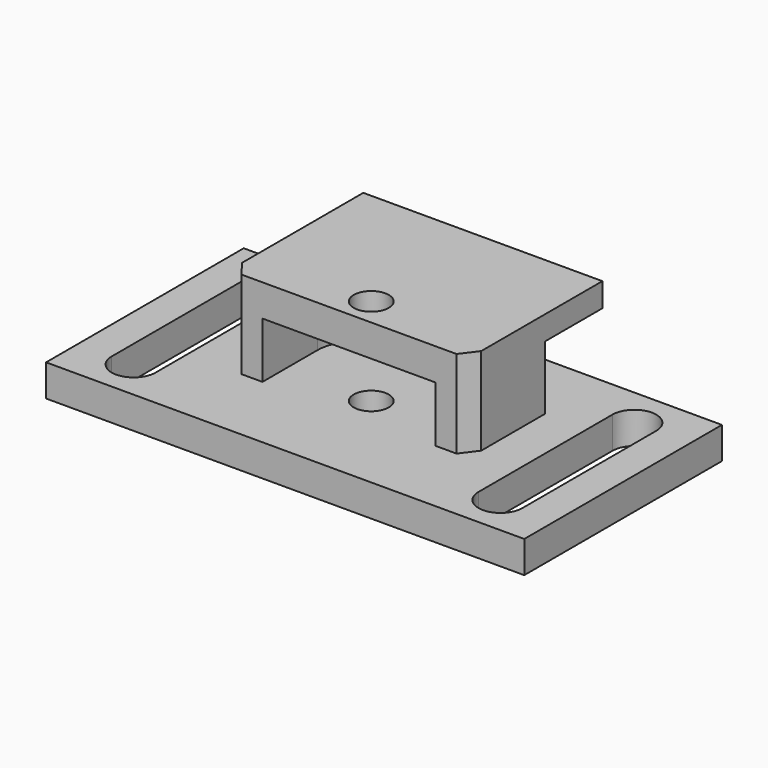
from build123d import *

# Parameters (mm, degrees)
F0_W         = 30
F0_H         = 26
F1_DEPTH     = 15
F3_SIZE2     = 2
F3_SIZE      = 1.5
F5_DEPTH     = 30.001
F6_SIZE      = 4
F2_W         = 21.7
F2_H         = 7
F7_DEPTH     = 12.5
F8_W         = 11
F8_H         = 7
F9_DEPTH     = 4
F10_W        = 30
F10_H        = 5
F11_DEPTH    = 15.001
F13_D        = 4.4
F15_DEPTH    = 4
F16_SIZE     = 3.49999
F17_T4_DEPTH = 26.4149188769
F18_SIZE     = 3.49999
F19_T4_DEPTH = 26.4149188769


# Not quite as in the source:
# - a fillet or chamfer that OpenCascade refuses, or shapes differently, is made with other operations: its cross-section is extruded or revolved along the edge and cut away or added
# - a fillet or chamfer is up to 0.001 mm smaller than in the source, because OpenCascade refuses the exact size


with BuildPart() as f1:
    # F0 (on Top) → F1 (new body)
    with BuildSketch(Plane.XY):
        Rectangle(F0_W, F0_H)
    extrude(amount=F1_DEPTH)

    # F3
    f3_edges = [f1.edges().sort_by_distance(p)[0] for p in [
        (-15, -13, 7.5),
        (15, -13, 7.5),
    ]]
    f3_side = f1.faces().sort_by_distance((0, -13, 7.5))[0]
    chamfer(f3_edges, length=F3_SIZE, length2=F3_SIZE2, reference=f3_side)

    # F4 (on face) → F5 (cut, through all)
    with BuildSketch(Plane(origin=(-15, 0, 0), x_dir=(0, -1, 0), z_dir=(-1, 0, 0))):
        Polygon((-13, 12), (-13, 0), (-8, 0), (-8, 4), (-3, 4), (-3, 12), align=None)
    extrude(amount=-F5_DEPTH, mode=Mode.SUBTRACT)

    # F6
    f6_edges = [f1.edges().sort_by_distance(p)[0] for p in [
        (-15, 3, 8),
        (15, 3, 8),
    ]]
    chamfer(f6_edges, length=F6_SIZE)

    # F2 (on face) → F7 (cut)
    with BuildSketch(Plane.XZ.offset(13)):
        with Locations((0, 7.5)):
            Rectangle(F2_W, F2_H)
    extrude(amount=-F7_DEPTH, mode=Mode.SUBTRACT)

    # F8 (on face) → F9 (cut)
    with BuildSketch(Plane(origin=(0, 3, 0), x_dir=(-1, 0, 0), z_dir=(0, 1, 0))):
        with Locations((0, 7.5)):
            Rectangle(F8_W, F8_H)
    extrude(amount=-F9_DEPTH, mode=Mode.SUBTRACT)

    # F10 (on face) → F11 (cut, through all)
    with BuildSketch(Plane.XY.offset(15)):
        with Locations((0, 10.5)):
            Rectangle(F10_W, F10_H)
    extrude(amount=-F11_DEPTH, mode=Mode.SUBTRACT)

    # F13 (through all)
    with Locations(Plane.XY.offset(15)):
        with Locations((0, -9.5)):
            Hole(F13_D / 2)

    # F14 (on face) → F15 (join)
    with BuildSketch(Plane(origin=(0, 0, 0), x_dir=(1, 0, 0), z_dir=(0, 0, -1))):
        with BuildLine():
            Line((30, 23), (-30, 23))
            Line((-30, 23), (-30, 11))
            Line((-30, 11), (-25.7624481171, 11))
            Line((-25.7624481171, 11), (-25.7624481171, 18))
            ThreePointArc((-25.7624481171, 18), (-23.0124481171, 20.75), (-20.2624481171, 18))
            Line((-20.2624481171, 18), (-20.2624481171, 11))
            Line((-20.2624481171, 11), (-15, 11))
            Line((-15, 11), (-13.5, 13))
            Line((-13.5, 13), (13.5, 13))
            Line((13.5, 13), (15, 11))
            Line((15, 11), (20.2624481171, 11))
            Line((20.2624481171, 11), (20.2624481171, 18))
            ThreePointArc((20.2624481171, 18), (23.0124481171, 20.75), (25.7624481171, 18))
            Line((25.7624481171, 18), (25.7624481171, 11))
            Line((25.7624481171, 11), (30, 11))
            Line((30, 11), (30, 23))
        make_face()
        with BuildLine():
            Line((-25.7624481171, 11), (-30, 11))
            Line((-30, 11), (-30, -8))
            Line((-30, -8), (-15, -8))
            Line((-15, -8), (-15, 11))
            Line((-15, 11), (-20.2624481171, 11))
            Line((-20.2624481171, 11), (-20.2624481171, -3))
            ThreePointArc((-20.2624481171, -3), (-23.0124481171, -5.75), (-25.7624481171, -3))
            Line((-25.7624481171, -3), (-25.7624481171, 11))
        make_face()
        with BuildLine():
            Line((30, -8), (30, 11))
            Line((30, 11), (25.7624481171, 11))
            Line((25.7624481171, 11), (25.7624481171, -3))
            ThreePointArc((25.7624481171, -3), (23.0124481171, -5.75), (20.2624481171, -3))
            Line((20.2624481171, -3), (20.2624481171, 11))
            Line((20.2624481171, 11), (15, 11))
            Line((15, 11), (15, -8))
            Line((15, -8), (30, -8))
        make_face()
    extrude(amount=-F15_DEPTH)

    # F16 (size 3.5 in the source; OpenCascade refuses exactly that, so slightly less here)
    f16_edges = [f1.edges().sort_by_distance(p)[0] for p in [
        (-5.5, -0.5, 7.5),
    ]]
    chamfer(f16_edges, length=F16_SIZE)

    # F17: fillet of radius 5 on 1 edges, made by hand


with BuildPart() as f17_tool2:
    # F17_s3 → F17_t4 (new body)
    with BuildSketch(Plane.XY.offset(20.7074594385)):
        with BuildLine():
            ThreePointArc((-8.99999, -0.5), (-10.3638647521, -2.2323966462), (-10.85, -4.3829837754))
            Line((-10.85, -4.3829837754), (-10.85, -0.5))
            Line((-10.85, -0.5), (-8.99999, -0.5))
        make_face()
    extrude(amount=-F17_T4_DEPTH)

    split(bisect_by=Plane.XY.offset(15), keep=Keep.BOTTOM)

    split(bisect_by=Plane.XY, keep=Keep.TOP)


with BuildPart() as f1_1:
    add(f1.part)

    # F17_t1: union F17_tool2
    add(f17_tool2.part)

    # F18 (size 3.5 in the source; OpenCascade refuses exactly that, so slightly less here)
    f18_edges = [f1_1.edges().sort_by_distance(p)[0] for p in [
        (5.5, -0.5, 7.5),
    ]]
    chamfer(f18_edges, length=F18_SIZE)

    # F19: fillet of radius 5 on 1 edges, made by hand


with BuildPart() as f19_tool2:
    # F19_s3 → F19_t4 (new body)
    with BuildSketch(Plane.XY.offset(-5.7074594385)):
        with BuildLine():
            ThreePointArc((8.99999, -0.5), (10.3638647521, -2.2323966462), (10.85, -4.3829837754))
            Line((10.85, -4.3829837754), (10.85, -0.5))
            Line((10.85, -0.5), (8.99999, -0.5))
        make_face()
    extrude(amount=F19_T4_DEPTH)

    split(bisect_by=Plane.XY.offset(15), keep=Keep.BOTTOM)

    split(bisect_by=Plane.XY, keep=Keep.TOP)


with BuildPart() as f1_2:
    add(f1_1.part)

    # F19_t1: union F19_tool2
    add(f19_tool2.part)


solid = f1_2.part
